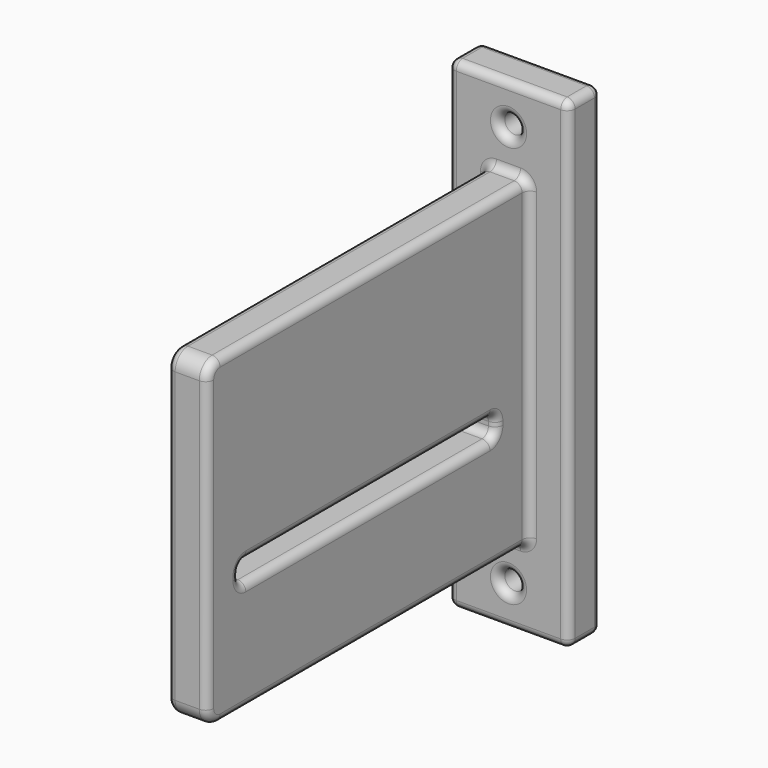
from build123d import *

# Parameters (mm, degrees)
F0_W     = 50
F0_H     = 40
F0_W_2   = 40
F0_H_2   = 2.5
F1_DEPTH = 2.5
F2_R     = 1
F3_R     = 2
F4_W     = 15
F4_H     = 60
F4_R     = 1.25
F4_W_2   = 5
F4_H_2   = 40
F5_DEPTH = 5
F6_DEPTH = 0.0001
F7_R     = 1


with BuildPart() as f1:
    # F0 (on Right) → F1 (new body, symmetric)
    with BuildSketch(Plane.YZ):
        Rectangle(F0_W, F0_H)
        with Locations((0, -5)):
            Rectangle(F0_W_2, F0_H_2, mode=Mode.SUBTRACT)
    extrude(amount=F1_DEPTH, both=True)

    # F2
    f2_edges = [f1.edges().sort_by_distance(p)[0] for p in [
        (0, -20, -6.25),
        (0, 20, -6.25),
        (0, 20, -3.75),
        (0, -20, -3.75),
    ]]
    fillet(f2_edges, radius=F2_R)

    # F3
    f3_edges = [f1.edges().sort_by_distance(p)[0] for p in [
        (0, -25, 20),
        (0, -25, -20),
    ]]
    fillet(f3_edges, radius=F3_R)

    # F4 (on face) → F5 (join)
    with BuildSketch(Plane(origin=(0, 25, 0), x_dir=(-1, 0, 0), z_dir=(0, 1, 0))):
        Rectangle(F4_W, F4_H)
        with Locations((0, -25)):
            Circle(F4_R, mode=Mode.SUBTRACT)
        Rectangle(F4_W_2, F4_H_2, mode=Mode.SUBTRACT)
        with Locations((0, 25)):
            Circle(F4_R, mode=Mode.SUBTRACT)
    extrude(amount=F5_DEPTH)

    # F4 (on face) → F6 (join)
    with BuildSketch(Plane(origin=(0, 25, 0), x_dir=(-1, 0, 0), z_dir=(0, 1, 0))):
        Rectangle(F4_W, F4_H)
        with Locations((0, -25)):
            Circle(F4_R, mode=Mode.SUBTRACT)
        with Locations((0, 25)):
            Circle(F4_R, mode=Mode.SUBTRACT)
    extrude(amount=F6_DEPTH)

    # F7
    f7_edges = [f1.edges().sort_by_distance(p)[0] for p in [
        (2.5, -25, 0),
        (2.5, -24.414214, 19.414214),
        (2.5, -24.414214, -19.414214),
        (2.5, 1, 20),
        (2.5, 1, -20),
        (2.5, 25, 0),
        (2.5, 0, -6.25),
        (2.5, 19.707107, -5.957107),
        (2.5, -19.707107, -5.957107),
        (2.5, 20, -5),
        (2.5, -20, -5),
        (2.5, 19.707107, -4.042893),
        (2.5, -19.707107, -4.042893),
        (2.5, 0, -3.75),
        (7.5, 25, 0),
        (0, 25, -30),
        (-7.5, 25, 0),
        (0, 25, 30),
        (1.25, 25, -25),
        (0, 25, -20),
        (0, 25, 20),
        (-2.5, 25, 0),
        (1.25, 25, 25),
        (-2.5, -25, 0),
        (-2.5, -24.414214, 19.414214),
        (-2.5, -24.414214, -19.414214),
        (-2.5, 1, 20),
        (-2.5, 1, -20),
        (-2.5, 0, -6.25),
        (-2.5, 19.707107, -5.957107),
        (-2.5, -19.707107, -5.957107),
        (-2.5, 20, -5),
        (-2.5, -20, -5),
        (-2.5, 19.707107, -4.042893),
        (-2.5, -19.707107, -4.042893),
        (-2.5, 0, -3.75),
        (-7.5, 27.5, -30),
        (-7.5, 30, 0),
        (-7.5, 27.5, 30),
        (7.5, 30, 0),
        (0, 30, -30),
        (0, 30, 30),
        (7.5, 27.5, 30),
        (7.5, 27.5, -30),
    ]]
    fillet(f7_edges, radius=F7_R)


solid = f1.part
